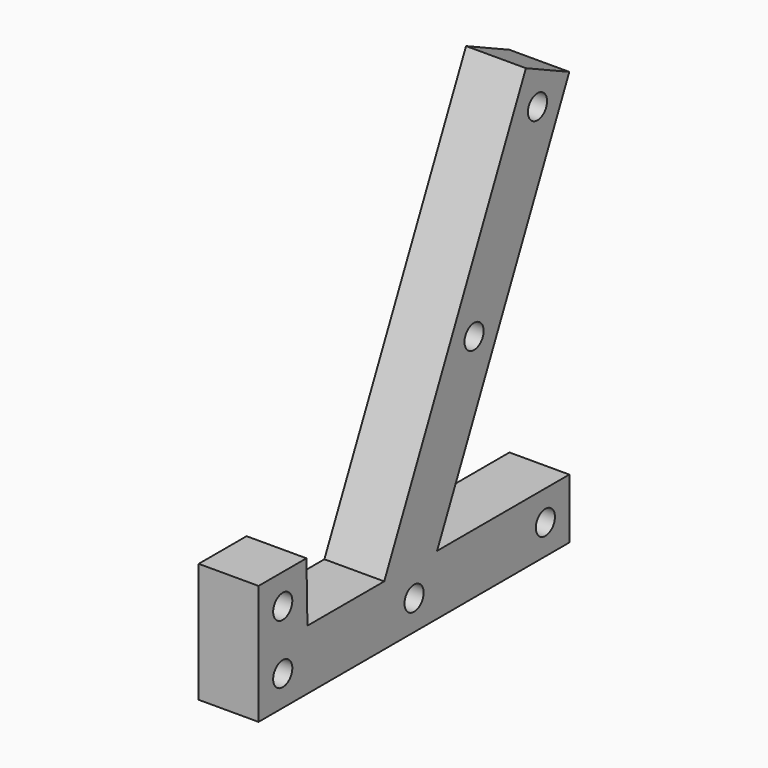
from build123d import *

# Parameters (mm, degrees)
F1_DEPTH = 10
F3_D     = 4
F3_DEPTH = 12
F3_TIP   = 1.2017212381


# Not quite as in the source:
# - a feature names something its author has since deleted; it is built from what else it names


with BuildPart() as f1:
    # F0 (on Right) → F1 (new body)
    with BuildSketch(Plane.YZ):
        Polygon((22.9933855712, -5), (22.9933855712, 5), (-4.6191914314, 5), (22.9933855712, 64.2153624752), (13.9303077009, 68.4415450926), (-15.652970621, 5), (-31.6901920953, 5), (-31.8974178605, 15), (-41.8974178605, 15), (-41.8974178605, -5), align=None)
    extrude(amount=F1_DEPTH)

    # F3
    with Locations(Plane.YZ.offset(10)):
        with Locations((16.3487553273, 61.7969148487), (17.9933855712, 0), (-9.4260048308, 0), (-36.8453457878, 0.0520720727), (3.1063371506, 33.3984574243), (-36.8456114192, 9.9481935587)):
            Hole(F3_D / 2, depth=F3_DEPTH)
            with Locations((0, 0, -(F3_DEPTH + F3_TIP / 2))):  # 118° drill point
                Cone(0, F3_D / 2, F3_TIP, mode=Mode.SUBTRACT)


solid = f1.part
